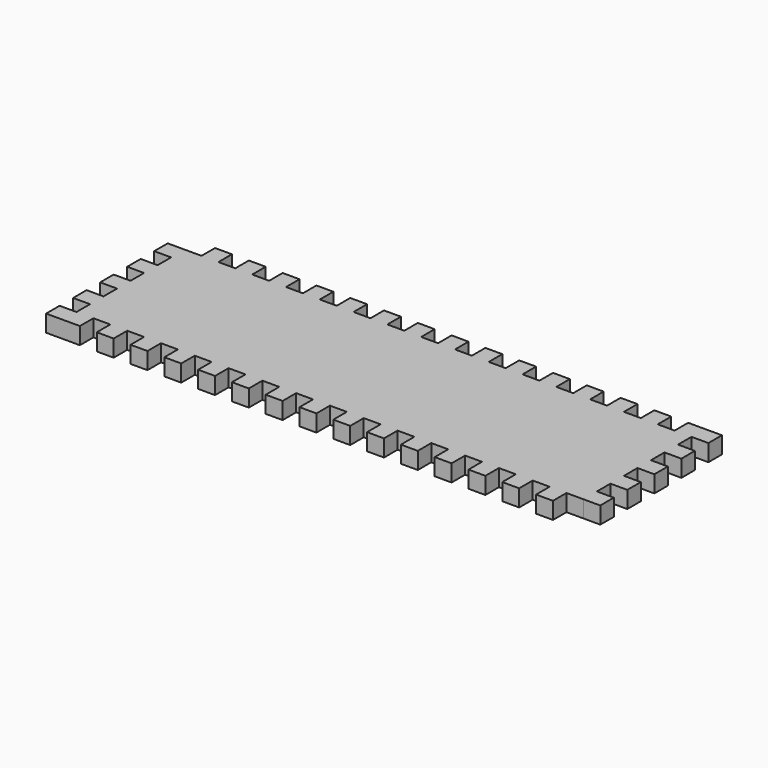
from build123d import *

# Parameters (mm, degrees)
F0_W     = 12.7
F0_H     = 12.7
F1_DEPTH = 12.7


# Not quite as in the source:
# - ends of sketch curves that miss each other by under 0.0002 mm in the source are joined
# - a feature names something its author has since deleted; it is built from what else it names


with BuildPart() as f1:
    # F0 (on Top) → F1 (new body)
    with BuildSketch(Plane.XY):
        Polygon((-112.6111072004, 68.7462910332), (-125.3111072004, 68.7462910332), (-125.3111072004, 56.0462910332), (-138.0111072004, 56.0462921858), (-138.0111072004, 43.3462910332), (-138.0111072004, 30.6462910332), (-138.0111072004, 17.9462910332), (-138.0111072004, 5.2462910332), (-138.0111072004, -7.4537089668), (-138.0111072004, -20.1537089668), (-138.0111072004, -32.8537089668), (-138.0111072004, -45.5537089668), (-138.0111072004, -58.2537089668), (-125.3111072004, -58.2537089668), (-125.3111072004, -45.5537089668), (-112.6111072004, -45.5537089668), (-112.6111072004, -58.2537089668), (-99.9111072004, -58.2537089668), (-99.9111072004, -45.5537089668), (-87.2111072004, -45.5537089668), (-87.2111072004, -58.2537089668), (-74.5111072004, -58.2537089668), (-74.5111072004, -45.5537089668), (-61.8111072004, -45.5537089668), (-61.8111072004, -58.2537089668), (-49.1111072004, -58.2537089668), (-49.1111072004, -45.5537089668), (-36.4111072004, -45.5537089668), (-36.4111072004, -58.2537089668), (-23.7111072004, -58.2537089668), (-23.7111072004, -45.5537089668), (-11.0111072004, -45.5537089668), (-11.0111072004, -58.2537089668), (1.6888927996, -58.2537089668), (1.6888927996, -45.5537089668), (14.3888927996, -45.5537089668), (14.3888927996, -58.2537089668), (27.0888927996, -58.2537089668), (27.0888927996, -45.5537089668), (39.7888927996, -45.5537089668), (39.7888927996, -58.2537089668), (52.4888927996, -58.2537089668), (52.4888927996, -45.5537089668), (65.1888927996, -45.5537089668), (65.1888927996, -58.2537089668), (77.8888927996, -58.2537089668), (77.8888927996, -45.5537089668), (90.5888927996, -45.5537089668), (90.5888927996, -58.2537089668), (103.2888927996, -58.2537089668), (103.2888927996, -45.5537089668), (115.9888927996, -45.5537089668), (115.9888927996, -58.2537089668), (128.6888927996, -58.2537089668), (128.6888927996, -45.5537089668), (141.3888927996, -45.5537089668), (141.3888927996, -58.2537089668), (154.0888927996, -58.2537089668), (154.0888927996, -45.5537089668), (166.7888927996, -45.5537089668), (166.7888927996, -58.2537089668), (179.4888927996, -58.2537089668), (179.4888927996, -45.5537089668), (192.1888927996, -45.5537089668), (192.1888927996, -58.2537089668), (204.8888927996, -58.2537089668), (204.8888927996, -45.5537089668), (217.5888927996, -45.5537089668), (217.5888927996, -58.2537089668), (230.2888927996, -58.2537089668), (230.2888927996, -45.5537089668), (242.9888927996, -45.5537089668), (242.9888927996, -32.8537103117), (242.9888927996, -20.1537098634), (242.9888927996, -7.4537103117), (242.9888927996, 5.2462896883), (242.9888927996, 17.9462896883), (242.9888927996, 30.6462901366), (242.9888927996, 43.3462896883), (242.9888927996, 56.0462905208), (242.9888927996, 68.7462910332), (230.2888927996, 68.7462910332), (230.2888927996, 56.0462921858), (217.5888927996, 56.0462921858), (217.5888927996, 68.7462921858), (204.8888927996, 68.7462910332), (204.8888927996, 56.0462921858), (192.1888927996, 56.0462921858), (192.1888927996, 68.7462910332), (179.4888927996, 68.7462910332), (179.4888927996, 56.0462921858), (166.7888927996, 56.0462921858), (166.7888927996, 68.7462921858), (154.0888927996, 68.7462910332), (154.0888927996, 56.0462921858), (141.3888927996, 56.0462921858), (141.3888927996, 68.7462910332), (128.6888927996, 68.7462910332), (128.6888927996, 56.0462921858), (115.9888927996, 56.0462921858), (115.9888927996, 68.7462921858), (103.2888927996, 68.7462910332), (103.2888927996, 56.0462921858), (90.5888927996, 56.0462921858), (90.5888927996, 68.7462921858), (77.8888927996, 68.7462910332), (77.8888927996, 56.0462921858), (65.1888927996, 56.0462921858), (65.1888927996, 68.7462921858), (52.4888927996, 68.7462910332), (52.4888927996, 56.0462921858), (39.7888927996, 56.0462921858), (39.7888927996, 68.7462921858), (27.0888927996, 68.7462910332), (27.0888927996, 56.0462921858), (14.3888927996, 56.0462921858), (14.3888927996, 68.7462921858), (1.6888927996, 68.7462910332), (1.6888927996, 56.0462921858), (-11.0111072004, 56.0462921858), (-11.0111072004, 68.7462921858), (-23.7111072004, 68.7462910332), (-23.7111072004, 56.0462921858), (-36.4111072004, 56.0462921858), (-36.4111072004, 68.7462921858), (-49.1111072004, 68.7462910332), (-49.1111072004, 56.0462921858), (-61.8111072004, 56.0462921858), (-61.8111072004, 68.7462921858), (-74.5111072004, 68.7462910332), (-74.5111072004, 56.0462921858), (-87.2111072004, 56.0462921858), (-87.2111072004, 68.7462921858), (-99.9111072004, 68.7462910332), (-99.9111072004, 56.0462921858), (-112.6111072004, 56.0462921858), align=None)
        with Locations((-144.3611072004, -51.9037089668)):
            Rectangle(F0_W, F0_H)
        Polygon((-138.0111072004, 43.3462910332), (-138.0111072004, 56.0462916095), (-150.7111072004, 56.0462910332), (-150.7111072004, 43.3462910332), align=None)
        with Locations((-144.3611072004, 24.2962910332)):
            Rectangle(F0_W, F0_H)
        with Locations((-144.3611072004, -1.1037089668)):
            Rectangle(F0_W, F0_H)
        with Locations((-144.3611072004, -26.5037089668)):
            Rectangle(F0_W, F0_H)
        with Locations((249.3388927996, -39.2037103117)):
            Rectangle(F0_W, F0_H)
        with Locations((249.3388927996, -13.8037103117)):
            Rectangle(F0_W, F0_H)
        with Locations((249.3388927996, 11.5962896883)):
            Rectangle(F0_W, F0_H)
        with Locations((249.3388927996, 36.9962896883)):
            Rectangle(F0_W, F0_H)
        Polygon((255.6888927996, 68.7462896883), (242.9888927996, 68.7462896883), (242.9888927996, 56.0462905208), (255.6888927996, 56.0462896883), align=None)
    extrude(amount=F1_DEPTH)


solid = f1.part
